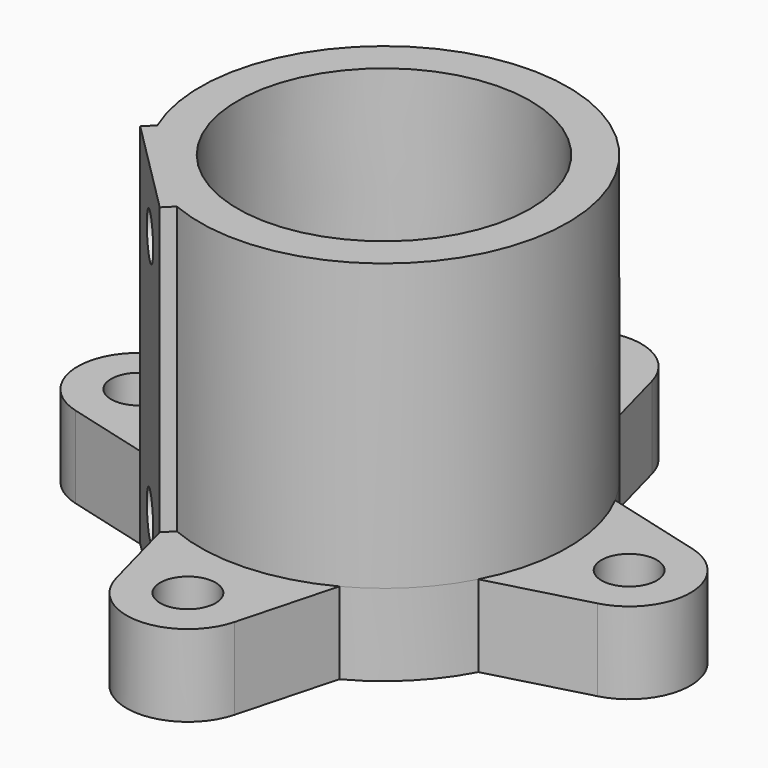
from build123d import *

# Parameters (mm, degrees)
F0_R     = 2.15265
F0_R_2   = 11.1125
F1_DEPTH = 6.35
F2_R     = 14.2875
F2_R_2   = 11.1125
F3_DEPTH = 22.225
F5_DEPTH = 28.575
F6_R     = 1.7272
F7_DEPTH = 4.3100488316


# Not quite as in the source:
# - a fillet or chamfer that OpenCascade refuses, or shapes differently, is made with other operations: its cross-section is extruded or revolved along the edge and cut away or added


with BuildPart() as f1:
    # F0 (on Top) → F1 (new body)
    with BuildSketch(Plane.XY):
        with BuildLine():
            Line((6.6460049492, 12.6476588531), (4.6002217477, 20.2826257023))
            ThreePointArc((4.6002217477, 20.2826257023), (0, 23.8125), (-4.6002217477, 20.2826257023))
            Line((-4.6002217477, 20.2826257023), (-6.6460049492, 12.6476588531))
            ThreePointArc((-6.6460049492, 12.6476588531), (-10.1027881362, 10.1027881362), (-12.6476588531, 6.6460049492))
            Line((-12.6476588531, 6.6460049492), (-20.2826257023, 4.6002217477))
            ThreePointArc((-20.2826257023, 4.6002217477), (-23.8125, 0), (-20.2826257023, -4.6002217477))
            Line((-20.2826257023, -4.6002217477), (-12.6476588531, -6.6460049492))
            ThreePointArc((-12.6476588531, -6.6460049492), (-10.1027881362, -10.1027881362), (-6.6460049492, -12.6476588531))
            Line((-6.6460049492, -12.6476588531), (-4.6002217477, -20.2826257023))
            ThreePointArc((-4.6002217477, -20.2826257023), (0, -23.8125), (4.6002217477, -20.2826257023))
            Line((4.6002217477, -20.2826257023), (6.6460049492, -12.6476588531))
            ThreePointArc((6.6460049492, -12.6476588531), (10.1027881362, -10.1027881362), (12.6476588531, -6.6460049492))
            Line((12.6476588531, -6.6460049492), (20.2826257023, -4.6002217477))
            ThreePointArc((20.2826257023, -4.6002217477), (23.8125, 0), (20.2826257023, 4.6002217477))
            Line((20.2826257023, 4.6002217477), (12.6476588531, 6.6460049492))
            ThreePointArc((12.6476588531, 6.6460049492), (10.1027881362, 10.1027881362), (6.6460049492, 12.6476588531))
        make_face()
        with Locations((0, -19.05)):
            Circle(F0_R, mode=Mode.SUBTRACT)
        with Locations((-19.05, 0)):
            Circle(F0_R, mode=Mode.SUBTRACT)
        Circle(F0_R_2, mode=Mode.SUBTRACT)
        with Locations((19.05, 0)):
            Circle(F0_R, mode=Mode.SUBTRACT)
        with Locations((0, 19.05)):
            Circle(F0_R, mode=Mode.SUBTRACT)
    extrude(amount=F1_DEPTH)

    # F2 (on face) → F3 (join)
    with BuildSketch(Plane.XY.offset(6.35)):
        Circle(F2_R)
        Circle(F2_R_2, mode=Mode.SUBTRACT)
    extrude(amount=F3_DEPTH)

    # F4 (on face) → F5 (join, through all)
    with BuildSketch(Plane.XY.offset(28.575)):
        Polygon((-4.0671577888, -11.648290423), (-11.648290423, -4.0671577888), (-13.8933544533, -6.3122218191), (-6.3122218191, -13.8933544533), align=None)
    extrude(amount=-F5_DEPTH)

    # F6 (on face) → F7 (cut, up to face)
    with BuildSketch(Plane(origin=(-10.1027881362, -10.1027881362, 0), x_dir=(0.7071067812, -0.7071067812, 0), z_dir=(-0.7071067812, -0.7071067812, 0))):
        with Locations((0, 23.8125)):
            Circle(F6_R)
        with Locations((0, 4.7625)):
            Circle(F6_R)
    extrude(amount=-F7_DEPTH, mode=Mode.SUBTRACT)

    # F8: chamfer of 28.575 x 0.254 on 1 edges, made by hand

    # F8_s1 → F8_t2 (revolve, cut)
    with BuildSketch(Plane.XZ):
        Polygon((11.3665, 28.575), (11.1125, 0), (11.1125, 28.575), align=None)
    revolve(axis=Axis((0, 0, 28.575), (0, 0, -1)), mode=Mode.SUBTRACT)


solid = f1.part
